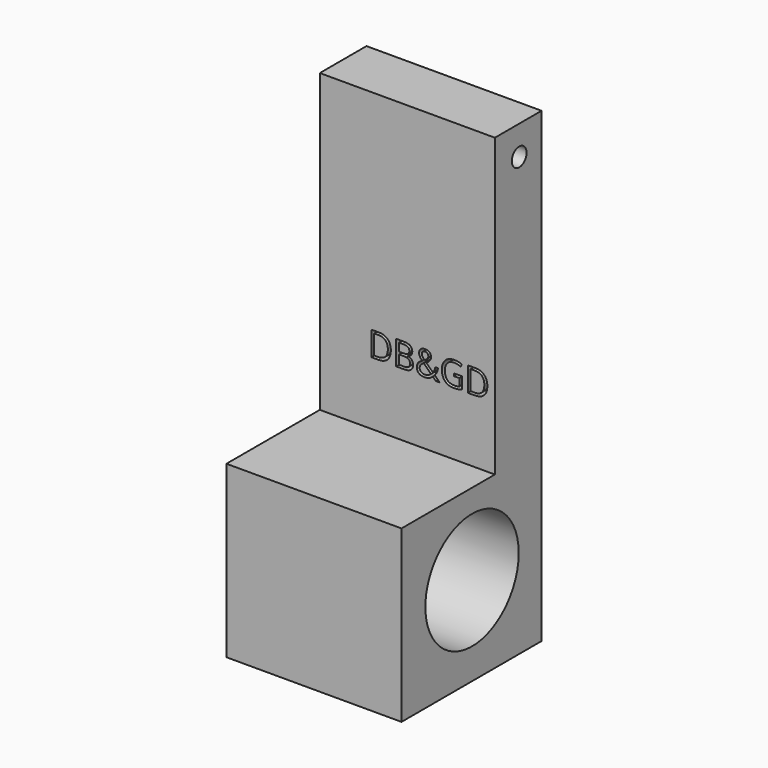
from build123d import *

# Parameters (mm, degrees)
F0_W         = 38.1
F0_H         = 101.6
F1_DEPTH     = 12.7
F2_W         = 38.1
F2_H         = 37.0723244905
F3_DEPTH     = 25.4
F4_R         = 12.7
F5_DEPTH     = 38.101
F7_R         = 2
F8_DEPTH     = 38.101
F9_TEXT_SIZE = 7.4083333333
F10_DEPTH    = 2.54


# Not quite as in the source:
# - Text() gives the source's letters only with a copy of the font that has no kerning and outlines rounded to 1/6400 em; it was checked with that copy


with BuildPart() as f1:
    # F0 (on Front) → F1 (new body)
    with BuildSketch(Plane.XZ):
        Rectangle(F0_W, F0_H)
    extrude(amount=F1_DEPTH)

    # F2 (on face) → F3 (join)
    with BuildSketch(Plane.XZ.offset(12.7)):
        with Locations((0, -32.2638377547)):
            Rectangle(F2_W, F2_H)
    extrude(amount=F3_DEPTH)

    # F4 (on face) → F5 (cut, through all)
    with BuildSketch(Plane.YZ.offset(19.05)):
        with Locations((-18.9130865037, -31.4218662679)):
            Circle(F4_R)
    extrude(amount=-F5_DEPTH, mode=Mode.SUBTRACT)

    # F7 (on face) → F8 (cut, through all)
    with BuildSketch(Plane(origin=(-19.05, 0, 0), x_dir=(0, -1, 0), z_dir=(-1, 0, 0))):
        with Locations((6.0837101191, 44.4295145571)):
            Circle(F7_R)
    extrude(amount=-F8_DEPTH, mode=Mode.SUBTRACT)

    # F9 (on face) → F10 (cut)
    with BuildSketch(Plane.XZ.offset(12.7)):
        with Locations((-8.5458708805, 0)):
            Text('DB&GD', F9_TEXT_SIZE, font='Open Sans', text_align=(TextAlign.LEFT, TextAlign.BOTTOM))
    extrude(amount=-F10_DEPTH, mode=Mode.SUBTRACT)


solid = f1.part
